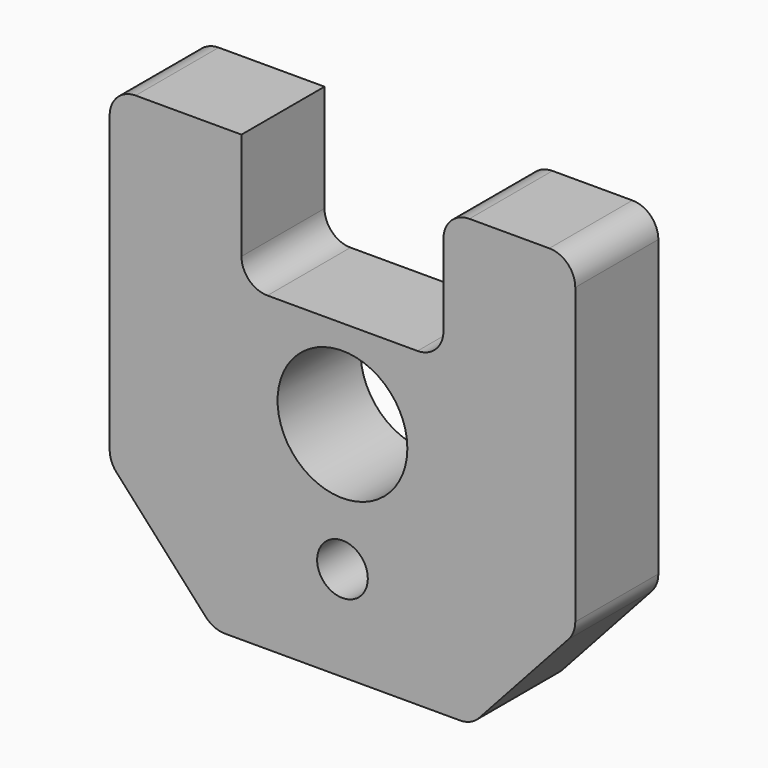
from build123d import *

# Parameters (mm, degrees)
F0_R     = 4.8825627193
F0_R_2   = 12.5
F1_DEPTH = 20
F2_R     = 5


with BuildPart() as f1:
    # F0 (on Front) → F1 (new body)
    with BuildSketch(Plane.XZ):
        with BuildLine():
            Line((-24.8438301682, -42.8251363337), (24.8438301682, -42.8251363337))
            Line((24.8438301682, -42.8251363337), (44.8438301682, -20.8251363337))
            Line((44.8438301682, -20.8251363337), (44.8438301682, 42.8251363337))
            Line((44.8438301682, 42.8251363337), (19.4535404444, 42.8251363337))
            Line((19.4535404444, 42.8251363337), (19.4535404444, 22.1680208296))
            ThreePointArc((19.4535404444, 22.1680208296), (17.9890743503, 18.6324869236), (14.4535404444, 17.1680208296))
            Line((14.4535404444, 17.1680208296), (-14.4535404444, 17.1680208296))
            ThreePointArc((-14.4535404444, 17.1680208296), (-17.9890743503, 18.6324869236), (-19.4535404444, 22.1680208296))
            Line((-19.4535404444, 22.1680208296), (-19.4535404444, 42.8251363337))
            Line((-19.4535404444, 42.8251363337), (-44.8438301682, 42.8251363337))
            Line((-44.8438301682, 42.8251363337), (-44.8438301682, -20.8251363337))
            Line((-44.8438301682, -20.8251363337), (-24.8438301682, -42.8251363337))
        make_face()
        with Locations((0, -24.5446097106)):
            Circle(F0_R, mode=Mode.SUBTRACT)
        Circle(F0_R_2, mode=Mode.SUBTRACT)
    extrude(amount=F1_DEPTH)

    # F2
    f2_edges = [f1.edges().sort_by_distance(p)[0] for p in [
        (44.84383, -10, 42.825136),
        (-24.84383, -10, -42.825136),
        (24.84383, -10, -42.825136),
        (44.84383, -10, -20.825136),
        (19.45354, -10, 42.825136),
        (-44.84383, -10, 42.825136),
        (-44.84383, -10, -20.825136),
    ]]
    fillet(f2_edges, radius=F2_R)


solid = f1.part
